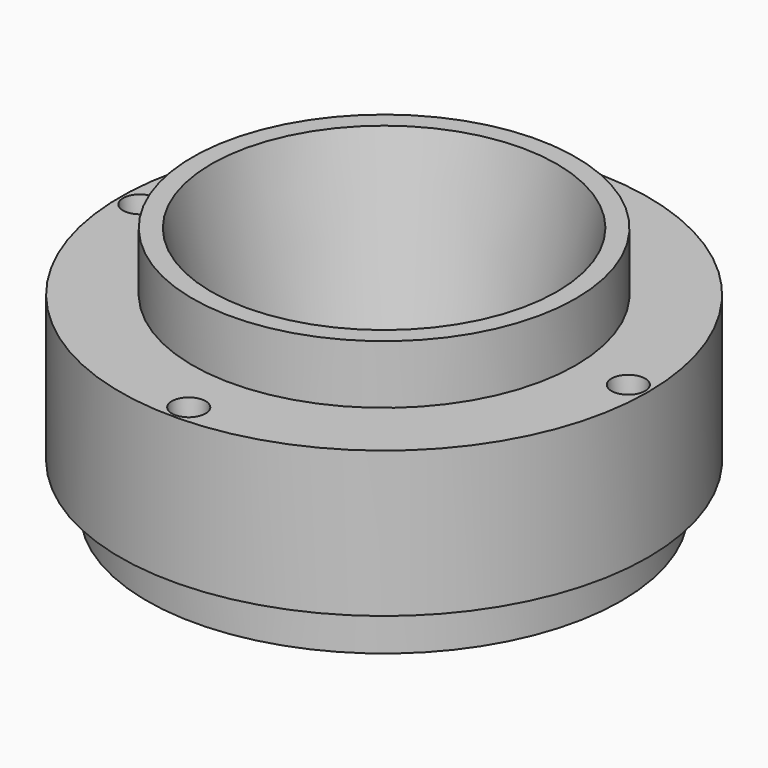
from build123d import *

# Parameters (mm, degrees)
F4_COPIES_COUNT = 4
F6_DEPTH        = 7


# Not quite as in the source:
# - a pattern or mirror of a feature is missing from the dataset's text; its kind, count and spacing are read off the source's solid


with BuildPart() as f1:
    # F0 (on Front) → F1 (revolve)
    with BuildSketch(Plane.XZ):
        Polygon((12.65, -40), (25.25, -40), (25.25, -35), (28.1, -35), (28.1, -19.5), (20.4, -19.5), (20.4, -13.25), (18.4, -13.25), (13.9, -37), (12.65, -37), align=None)
    revolve(axis=Axis((0, 0, -3.8875962891), (0, 0, -1)))

    # F3 (on Front) → F4 (revolve, cut)
    with BuildSketch(Plane.XZ):
        Polygon((27.7907, -19.5), (25.9972140193, -19.5), (25.9972140193, -22.421), (27.5621, -22.421), align=None)
    f4 = revolve(axis=Axis((25.9972140193, 0, -20.9605), (0, 0, 1)), mode=Mode.SUBTRACT)

    # F4_copies: F4 ×4 about axis
    f4_copies_axis = Axis((0, 0, 0), (0, 0, 1))
    for i in range(1, F4_COPIES_COUNT):
        add(f4.rotate(f4_copies_axis, i * 360 / F4_COPIES_COUNT), mode=Mode.SUBTRACT)

    # F5 (on face) → F6 (cut)
    with BuildSketch(Plane(origin=(0, 0, -40), x_dir=(1, 0, 0), z_dir=(0, 0, -1))):
        with BuildLine():
            Line((-3.5, 18.75), (-3.5, 15.15))
            Line((-3.5, 15.15), (3.5, 15.15))
            Line((3.5, 15.15), (3.5, 18.75))
            ThreePointArc((3.5, 18.75), (2.4748737342, 21.2248737342), (0, 22.25))
            ThreePointArc((0, 22.25), (-2.4748737342, 21.2248737342), (-3.5, 18.75))
        make_face()
        with BuildLine():
            ThreePointArc((23.25, 3), (22.6642135624, 4.4142135624), (21.25, 5))
            Line((21.25, 5), (16.15, 5))
            Line((16.15, 5), (16.15, -5))
            Line((16.15, -5), (21.25, -5))
            ThreePointArc((21.25, -5), (22.6642135624, -4.4142135624), (23.25, -3))
            Line((23.25, -3), (23.25, 3))
        make_face()
    extrude(amount=-F6_DEPTH, mode=Mode.SUBTRACT)


solid = f1.part
